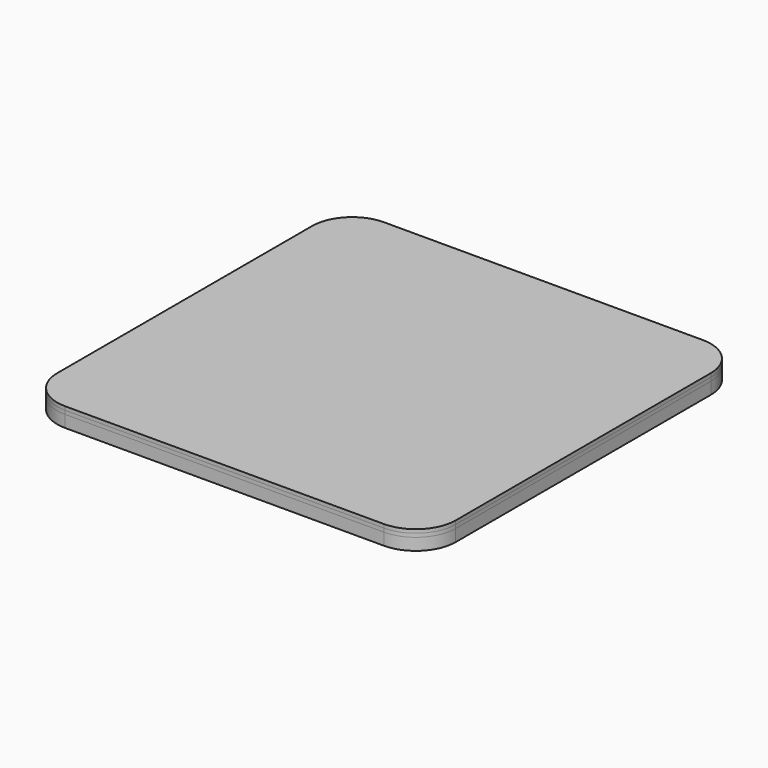
from build123d import *

# Parameters (mm, degrees)
F0_W     = 30
F0_H     = 30
F1_DEPTH = 0.27
F2_R     = 3
F3_DEPTH = 0.27
F4_DEPTH = 0.9
F5_W     = 24
F5_H     = 24
F6_DEPTH = 25
F7_DEPTH = 0.6
F8_DEPTH = 0.54


with BuildPart() as f1:
    # F0 (on Top) → F1 (new body)
    with BuildSketch(Plane.XY):
        with Locations((15, 15)):
            Rectangle(F0_W, F0_H)
    extrude(amount=F1_DEPTH)

    # F2
    f2_edges = [f1.edges().sort_by_distance(p)[0] for p in [
        (30, 0, 0.135),
        (30, 30, 0.135),
        (0, 30, 0.135),
        (0, 0, 0.135),
    ]]
    fillet(f2_edges, radius=F2_R)


with BuildPart() as f3:
    # F3 (new): a face of the model
    f3_faces = [f1.part.faces().sort_by_distance(p)[0] for p in [
        (15, 15, 0.27),
    ]]
    extrude(f3_faces, amount=F3_DEPTH)


with BuildPart() as f4:
    # F4 (new): a face of the model
    f4_faces = [f1.part.faces().sort_by_distance(p)[0] for p in [
        (15, 15, 0),
    ]]
    extrude(f4_faces, amount=F4_DEPTH)

    # F5 (on face) → F6 (cut)
    with BuildSketch(Plane(origin=(0, 0, -0.9), x_dir=(1, 0, 0), z_dir=(0, 0, -1))):
        with Locations((15, -15)):
            Rectangle(F5_W, F5_H)
    extrude(amount=-F6_DEPTH, mode=Mode.SUBTRACT)


with BuildPart() as f7:
    # F5 (on face) → F7 (new body)
    with BuildSketch(Plane(origin=(0, 0, -0.9), x_dir=(1, 0, 0), z_dir=(0, 0, -1))):
        with Locations((15, -15)):
            Rectangle(F5_W, F5_H)
    extrude(amount=F7_DEPTH)

    # F5 (on face) → F8 (join)
    with BuildSketch(Plane(origin=(0, 0, -0.9), x_dir=(1, 0, 0), z_dir=(0, 0, -1))):
        with Locations((15, -15)):
            Rectangle(F5_W, F5_H)
    extrude(amount=-F8_DEPTH)


solid = Compound([f1.part, f3.part, f4.part, f7.part])
